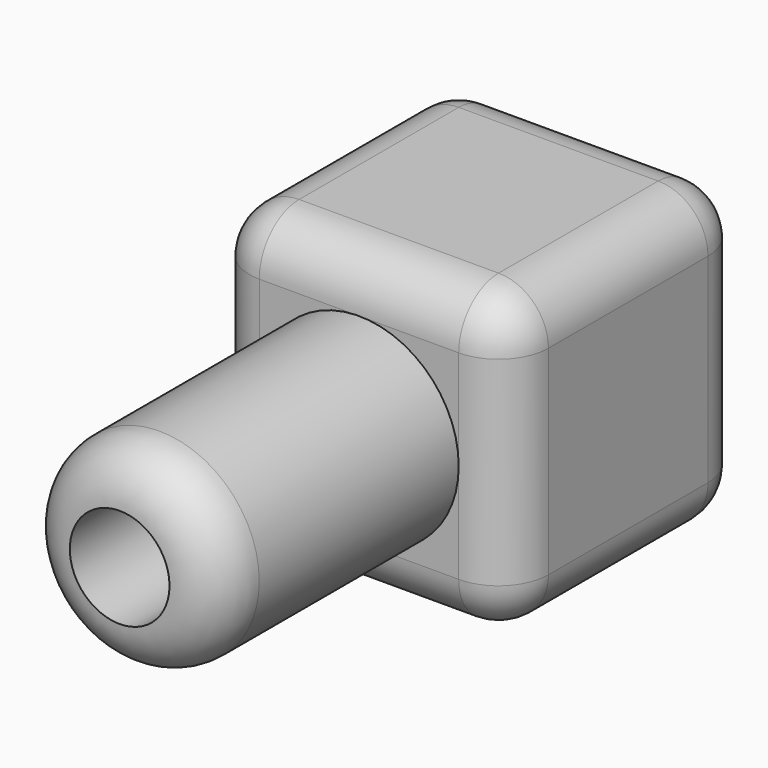
from build123d import *

# Parameters (mm, degrees)
F0_W     = 30
F0_H     = 30
F1_DEPTH = 30
F2_R     = 10
F3_DEPTH = 30
F4_R     = 5
F5_DEPTH = 60.001
F6_R     = 4.99999


# Not quite as in the source:
# - a fillet or chamfer is up to 0.001 mm smaller than in the source, because OpenCascade refuses the exact size


with BuildPart() as f1:
    # F0 (on Front) → F1 (new body)
    with BuildSketch(Plane.XZ):
        Rectangle(F0_W, F0_H)
    extrude(amount=F1_DEPTH)

    # F2 (on face) → F3 (join)
    with BuildSketch(Plane.XZ.offset(30)):
        Circle(F2_R)
    extrude(amount=F3_DEPTH)

    # F4 (on face) → F5 (cut, through all)
    with BuildSketch(Plane.XZ.offset(60)):
        Circle(F4_R)
    extrude(amount=-F5_DEPTH, mode=Mode.SUBTRACT)

    # F6 (radius 5 in the source; OpenCascade refuses exactly that, so slightly less here)
    f6_edges = [f1.edges().sort_by_distance(p)[0] for p in [
        (0, -30, 15),
        (-15, -30, 0),
        (0, -30, -15),
        (15, -30, 0),
        (15, -15, 15),
        (15, -15, -15),
        (0, 0, -15),
        (-15, 0, 0),
        (15, 0, 0),
        (0, 0, 15),
        (-15, -15, 15),
        (-10, -60, 0),
        (-15, -15, -15),
    ]]
    fillet(f6_edges, radius=F6_R)


solid = f1.part
